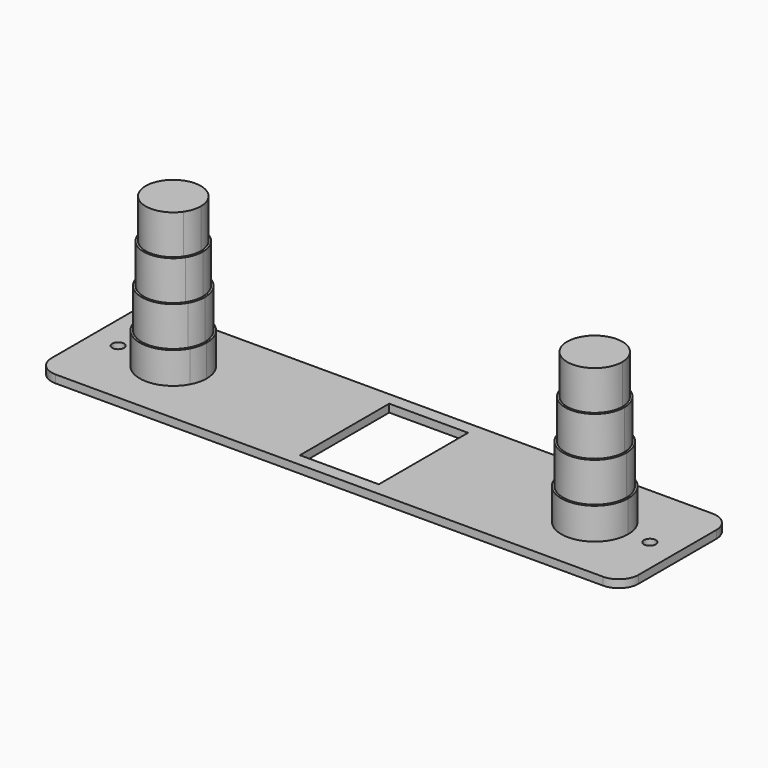
from build123d import *

# Parameters (mm, degrees)
F0_R     = 1.5
F1_DEPTH = 2
F2_DEPTH = 40
F3_DEPTH = 30
F4_DEPTH = 20
F5_DEPTH = 10


with BuildPart() as f1:
    # F0 (on Top) → F1 (new body)
    with BuildSketch(Plane.XY):
        with BuildLine():
            Line((69.5, 17.3640065603), (-69.5, 17.3640065603))
            ThreePointArc((-69.5, 17.3640065603), (-73.0355339059, 15.8995404662), (-74.5, 12.3640065603))
            Line((-74.5, 12.3640065603), (-74.5, -12.3640065603))
            ThreePointArc((-74.5, -12.3640065603), (-73.0355339059, -15.8995404662), (-69.5, -17.3640065603))
            Line((-69.5, -17.3640065603), (69.5, -17.3640065603))
            ThreePointArc((69.5, -17.3640065603), (73.0355339059, -15.8995404662), (74.5, -12.3640065603))
            Line((74.5, -12.3640065603), (74.5, 12.3640065603))
            ThreePointArc((74.5, 12.3640065603), (73.0355339059, 15.8995404662), (69.5, 17.3640065603))
        make_face()
        with Locations((-67.5, 0)):
            Circle(F0_R, mode=Mode.SUBTRACT)
        with BuildLine():
            ThreePointArc((-46, -4), (-62, 0), (-46, 4))
            Line((-46, 4), (-10.0108450279, 4))
            Line((-10.0108450279, 4), (-10.0108450279, 14.1616659239))
            Line((-10.0108450279, 14.1616659239), (10.0108450279, 14.1616659239))
            Line((10.0108450279, 14.1616659239), (10.0108450279, 4))
            Line((10.0108450279, 4), (46, 4))
            ThreePointArc((46, 4), (55.5615528128, 8.2462112512), (62, 0))
            ThreePointArc((62, 0), (55.5615528128, -8.2462112512), (46, -4))
            Line((46, -4), (10.0108450279, -4))
            Line((10.0108450279, -4), (10.0108450279, -14.1616659239))
            Line((10.0108450279, -14.1616659239), (-10.0108450279, -14.1616659239))
            Line((-10.0108450279, -14.1616659239), (-10.0108450279, -4))
            Line((-10.0108450279, -4), (-46, -4))
        make_face(mode=Mode.SUBTRACT)
        with Locations((67.5, 0)):
            Circle(F0_R, mode=Mode.SUBTRACT)
        with BuildLine():
            Line((-10.0108450279, 4), (-46, 4))
            ThreePointArc((-46, 4), (-45.2537887488, 2.0615528128), (-45, 0))
            ThreePointArc((-45, 0), (-45.2537887488, -2.0615528128), (-46, -4))
            Line((-46, -4), (-10.0108450279, -4))
            Line((-10.0108450279, -4), (-10.0108450279, 4))
        make_face()
        with BuildLine():
            Line((46, 4), (10.0108450279, 4))
            Line((10.0108450279, 4), (10.0108450279, -4))
            Line((10.0108450279, -4), (46, -4))
            ThreePointArc((46, -4), (45, 0), (46, 4))
        make_face()
        with BuildLine():
            ThreePointArc((-47.7554373535, -4), (-46.8212299588, -2.0961943462), (-46.5, 0))
            ThreePointArc((-46.5, 0), (-46.8212299588, 2.0961943462), (-47.7554373535, 4))
            Line((-47.7554373535, 4), (-53.5, 4))
            Line((-53.5, 4), (-53.5, -4))
            Line((-53.5, -4), (-47.7554373535, -4))
        make_face()
        with BuildLine():
            Line((-53.5, 4), (-47.7554373535, 4))
            ThreePointArc((-47.7554373535, 4), (-60.5, 0), (-47.7554373535, -4))
            Line((-47.7554373535, -4), (-53.5, -4))
            Line((-53.5, -4), (-53.5, 4))
        make_face()
        with BuildLine():
            ThreePointArc((-47.7554373535, -4), (-60.5, 0), (-47.7554373535, 4))
            Line((-47.7554373535, 4), (-47.1557112298, 4))
            ThreePointArc((-47.1557112298, 4), (-61, 0), (-47.1557112298, -4))
            Line((-47.1557112298, -4), (-47.7554373535, -4))
        make_face()
        with BuildLine():
            ThreePointArc((-47.1557112298, -4), (-61, 0), (-47.1557112298, 4))
            Line((-47.1557112298, 4), (-46.5717967697, 4))
            ThreePointArc((-46.5717967697, 4), (-61.5, 0), (-46.5717967697, -4))
            Line((-46.5717967697, -4), (-47.1557112298, -4))
        make_face()
        with BuildLine():
            ThreePointArc((-46.5717967697, -4), (-61.5, 0), (-46.5717967697, 4))
            Line((-46.5717967697, 4), (-46, 4))
            ThreePointArc((-46, 4), (-62, 0), (-46, -4))
            Line((-46, -4), (-46.5717967697, -4))
        make_face()
        with BuildLine():
            ThreePointArc((-47.7554373535, 4), (-46.8212299588, 2.0961943462), (-46.5, 0))
            ThreePointArc((-46.5, 0), (-46.8212299588, -2.0961943462), (-47.7554373535, -4))
            Line((-47.7554373535, -4), (-47.1557112298, -4))
            ThreePointArc((-47.1557112298, -4), (-46.2947184033, -2.0818062138), (-46, 0))
            ThreePointArc((-46, 0), (-46.2947184033, 2.0818062138), (-47.1557112298, 4))
            Line((-47.1557112298, 4), (-47.7554373535, 4))
        make_face()
        with BuildLine():
            Line((-46.5717967697, 4), (-47.1557112298, 4))
            ThreePointArc((-47.1557112298, 4), (-46.2947184033, 2.0818062138), (-46, 0))
            ThreePointArc((-46, 0), (-46.2947184033, -2.0818062138), (-47.1557112298, -4))
            Line((-47.1557112298, -4), (-46.5717967697, -4))
            ThreePointArc((-46.5717967697, -4), (-45.7725933897, -2.0705523608), (-45.5, 0))
            ThreePointArc((-45.5, 0), (-45.7725933897, 2.0705523608), (-46.5717967697, 4))
        make_face()
        with BuildLine():
            Line((-46, 4), (-46.5717967697, 4))
            ThreePointArc((-46.5717967697, 4), (-45.7725933897, 2.0705523608), (-45.5, 0))
            ThreePointArc((-45.5, 0), (-45.7725933897, -2.0705523608), (-46.5717967697, -4))
            Line((-46.5717967697, -4), (-46, -4))
            ThreePointArc((-46, -4), (-45.2537887488, -2.0615528128), (-45, 0))
            ThreePointArc((-45, 0), (-45.2537887488, 2.0615528128), (-46, 4))
        make_face()
        with BuildLine():
            ThreePointArc((60.5, 0), (55.5961943462, 6.6787700412), (47.7554373535, 4))
            Line((47.7554373535, 4), (53.5, 4))
            Line((53.5, 4), (53.5, -4))
            Line((53.5, -4), (47.7554373535, -4))
            ThreePointArc((47.7554373535, -4), (55.5961943462, -6.6787700412), (60.5, 0))
        make_face()
        with BuildLine():
            Line((53.5, 4), (47.7554373535, 4))
            ThreePointArc((47.7554373535, 4), (46.5, 0), (47.7554373535, -4))
            Line((47.7554373535, -4), (53.5, -4))
            Line((53.5, -4), (53.5, 4))
        make_face()
        with BuildLine():
            Line((47.7554373535, 4), (47.1557112298, 4))
            ThreePointArc((47.1557112298, 4), (46, 0), (47.1557112298, -4))
            Line((47.1557112298, -4), (47.7554373535, -4))
            ThreePointArc((47.7554373535, -4), (46.5, 0), (47.7554373535, 4))
        make_face()
        with BuildLine():
            Line((47.1557112298, 4), (46.5717967697, 4))
            ThreePointArc((46.5717967697, 4), (45.5, 0), (46.5717967697, -4))
            Line((46.5717967697, -4), (47.1557112298, -4))
            ThreePointArc((47.1557112298, -4), (46, 0), (47.1557112298, 4))
        make_face()
        with BuildLine():
            Line((46.5717967697, 4), (46, 4))
            ThreePointArc((46, 4), (45, 0), (46, -4))
            Line((46, -4), (46.5717967697, -4))
            ThreePointArc((46.5717967697, -4), (45.5, 0), (46.5717967697, 4))
        make_face()
        with BuildLine():
            ThreePointArc((62, 0), (55.5615528128, 8.2462112512), (46, 4))
            Line((46, 4), (46.5717967697, 4))
            ThreePointArc((46.5717967697, 4), (55.5705523608, 7.7274066103), (61.5, 0))
            ThreePointArc((61.5, 0), (55.5705523608, -7.7274066103), (46.5717967697, -4))
            Line((46.5717967697, -4), (46, -4))
            ThreePointArc((46, -4), (55.5615528128, -8.2462112512), (62, 0))
        make_face()
        with BuildLine():
            ThreePointArc((61.5, 0), (55.5705523608, 7.7274066103), (46.5717967697, 4))
            Line((46.5717967697, 4), (47.1557112298, 4))
            ThreePointArc((47.1557112298, 4), (55.5818062138, 7.2052815967), (61, 0))
            ThreePointArc((61, 0), (55.5818062138, -7.2052815967), (47.1557112298, -4))
            Line((47.1557112298, -4), (46.5717967697, -4))
            ThreePointArc((46.5717967697, -4), (55.5705523608, -7.7274066103), (61.5, 0))
        make_face()
        with BuildLine():
            ThreePointArc((61, 0), (55.5818062138, 7.2052815967), (47.1557112298, 4))
            Line((47.1557112298, 4), (47.7554373535, 4))
            ThreePointArc((47.7554373535, 4), (55.5961943462, 6.6787700412), (60.5, 0))
            ThreePointArc((60.5, 0), (55.5961943462, -6.6787700412), (47.7554373535, -4))
            Line((47.7554373535, -4), (47.1557112298, -4))
            ThreePointArc((47.1557112298, -4), (55.5818062138, -7.2052815967), (61, 0))
        make_face()
    extrude(amount=F1_DEPTH)

    # F0 (on Top) → F2 (join)
    with BuildSketch(Plane.XY):
        with BuildLine():
            Line((-53.5, 4), (-47.7554373535, 4))
            ThreePointArc((-47.7554373535, 4), (-60.5, 0), (-47.7554373535, -4))
            Line((-47.7554373535, -4), (-53.5, -4))
            Line((-53.5, -4), (-53.5, 4))
        make_face()
        with BuildLine():
            ThreePointArc((-47.7554373535, -4), (-46.8212299588, -2.0961943462), (-46.5, 0))
            ThreePointArc((-46.5, 0), (-46.8212299588, 2.0961943462), (-47.7554373535, 4))
            Line((-47.7554373535, 4), (-53.5, 4))
            Line((-53.5, 4), (-53.5, -4))
            Line((-53.5, -4), (-47.7554373535, -4))
        make_face()
        with BuildLine():
            Line((53.5, 4), (47.7554373535, 4))
            ThreePointArc((47.7554373535, 4), (46.5, 0), (47.7554373535, -4))
            Line((47.7554373535, -4), (53.5, -4))
            Line((53.5, -4), (53.5, 4))
        make_face()
        with BuildLine():
            ThreePointArc((60.5, 0), (55.5961943462, 6.6787700412), (47.7554373535, 4))
            Line((47.7554373535, 4), (53.5, 4))
            Line((53.5, 4), (53.5, -4))
            Line((53.5, -4), (47.7554373535, -4))
            ThreePointArc((47.7554373535, -4), (55.5961943462, -6.6787700412), (60.5, 0))
        make_face()
    extrude(amount=F2_DEPTH)

    # F0 (on Top) → F3 (join)
    with BuildSketch(Plane.XY):
        with BuildLine():
            ThreePointArc((-47.7554373535, -4), (-60.5, 0), (-47.7554373535, 4))
            Line((-47.7554373535, 4), (-47.1557112298, 4))
            ThreePointArc((-47.1557112298, 4), (-61, 0), (-47.1557112298, -4))
            Line((-47.1557112298, -4), (-47.7554373535, -4))
        make_face()
        with BuildLine():
            ThreePointArc((-47.7554373535, 4), (-46.8212299588, 2.0961943462), (-46.5, 0))
            ThreePointArc((-46.5, 0), (-46.8212299588, -2.0961943462), (-47.7554373535, -4))
            Line((-47.7554373535, -4), (-47.1557112298, -4))
            ThreePointArc((-47.1557112298, -4), (-46.2947184033, -2.0818062138), (-46, 0))
            ThreePointArc((-46, 0), (-46.2947184033, 2.0818062138), (-47.1557112298, 4))
            Line((-47.1557112298, 4), (-47.7554373535, 4))
        make_face()
        with BuildLine():
            Line((47.7554373535, 4), (47.1557112298, 4))
            ThreePointArc((47.1557112298, 4), (46, 0), (47.1557112298, -4))
            Line((47.1557112298, -4), (47.7554373535, -4))
            ThreePointArc((47.7554373535, -4), (46.5, 0), (47.7554373535, 4))
        make_face()
        with BuildLine():
            ThreePointArc((61, 0), (55.5818062138, 7.2052815967), (47.1557112298, 4))
            Line((47.1557112298, 4), (47.7554373535, 4))
            ThreePointArc((47.7554373535, 4), (55.5961943462, 6.6787700412), (60.5, 0))
            ThreePointArc((60.5, 0), (55.5961943462, -6.6787700412), (47.7554373535, -4))
            Line((47.7554373535, -4), (47.1557112298, -4))
            ThreePointArc((47.1557112298, -4), (55.5818062138, -7.2052815967), (61, 0))
        make_face()
    extrude(amount=F3_DEPTH)

    # F0 (on Top) → F4 (join)
    with BuildSketch(Plane.XY):
        with BuildLine():
            ThreePointArc((-47.1557112298, -4), (-61, 0), (-47.1557112298, 4))
            Line((-47.1557112298, 4), (-46.5717967697, 4))
            ThreePointArc((-46.5717967697, 4), (-61.5, 0), (-46.5717967697, -4))
            Line((-46.5717967697, -4), (-47.1557112298, -4))
        make_face()
        with BuildLine():
            Line((-46.5717967697, 4), (-47.1557112298, 4))
            ThreePointArc((-47.1557112298, 4), (-46.2947184033, 2.0818062138), (-46, 0))
            ThreePointArc((-46, 0), (-46.2947184033, -2.0818062138), (-47.1557112298, -4))
            Line((-47.1557112298, -4), (-46.5717967697, -4))
            ThreePointArc((-46.5717967697, -4), (-45.7725933897, -2.0705523608), (-45.5, 0))
            ThreePointArc((-45.5, 0), (-45.7725933897, 2.0705523608), (-46.5717967697, 4))
        make_face()
        with BuildLine():
            Line((47.1557112298, 4), (46.5717967697, 4))
            ThreePointArc((46.5717967697, 4), (45.5, 0), (46.5717967697, -4))
            Line((46.5717967697, -4), (47.1557112298, -4))
            ThreePointArc((47.1557112298, -4), (46, 0), (47.1557112298, 4))
        make_face()
        with BuildLine():
            ThreePointArc((61.5, 0), (55.5705523608, 7.7274066103), (46.5717967697, 4))
            Line((46.5717967697, 4), (47.1557112298, 4))
            ThreePointArc((47.1557112298, 4), (55.5818062138, 7.2052815967), (61, 0))
            ThreePointArc((61, 0), (55.5818062138, -7.2052815967), (47.1557112298, -4))
            Line((47.1557112298, -4), (46.5717967697, -4))
            ThreePointArc((46.5717967697, -4), (55.5705523608, -7.7274066103), (61.5, 0))
        make_face()
    extrude(amount=F4_DEPTH)

    # F0 (on Top) → F5 (join)
    with BuildSketch(Plane.XY):
        with BuildLine():
            Line((46.5717967697, 4), (46, 4))
            ThreePointArc((46, 4), (45, 0), (46, -4))
            Line((46, -4), (46.5717967697, -4))
            ThreePointArc((46.5717967697, -4), (45.5, 0), (46.5717967697, 4))
        make_face()
        with BuildLine():
            ThreePointArc((62, 0), (55.5615528128, 8.2462112512), (46, 4))
            Line((46, 4), (46.5717967697, 4))
            ThreePointArc((46.5717967697, 4), (55.5705523608, 7.7274066103), (61.5, 0))
            ThreePointArc((61.5, 0), (55.5705523608, -7.7274066103), (46.5717967697, -4))
            Line((46.5717967697, -4), (46, -4))
            ThreePointArc((46, -4), (55.5615528128, -8.2462112512), (62, 0))
        make_face()
        with BuildLine():
            Line((-46, 4), (-46.5717967697, 4))
            ThreePointArc((-46.5717967697, 4), (-45.7725933897, 2.0705523608), (-45.5, 0))
            ThreePointArc((-45.5, 0), (-45.7725933897, -2.0705523608), (-46.5717967697, -4))
            Line((-46.5717967697, -4), (-46, -4))
            ThreePointArc((-46, -4), (-45.2537887488, -2.0615528128), (-45, 0))
            ThreePointArc((-45, 0), (-45.2537887488, 2.0615528128), (-46, 4))
        make_face()
        with BuildLine():
            ThreePointArc((-46.5717967697, -4), (-61.5, 0), (-46.5717967697, 4))
            Line((-46.5717967697, 4), (-46, 4))
            ThreePointArc((-46, 4), (-62, 0), (-46, -4))
            Line((-46, -4), (-46.5717967697, -4))
        make_face()
    extrude(amount=F5_DEPTH)


solid = f1.part
